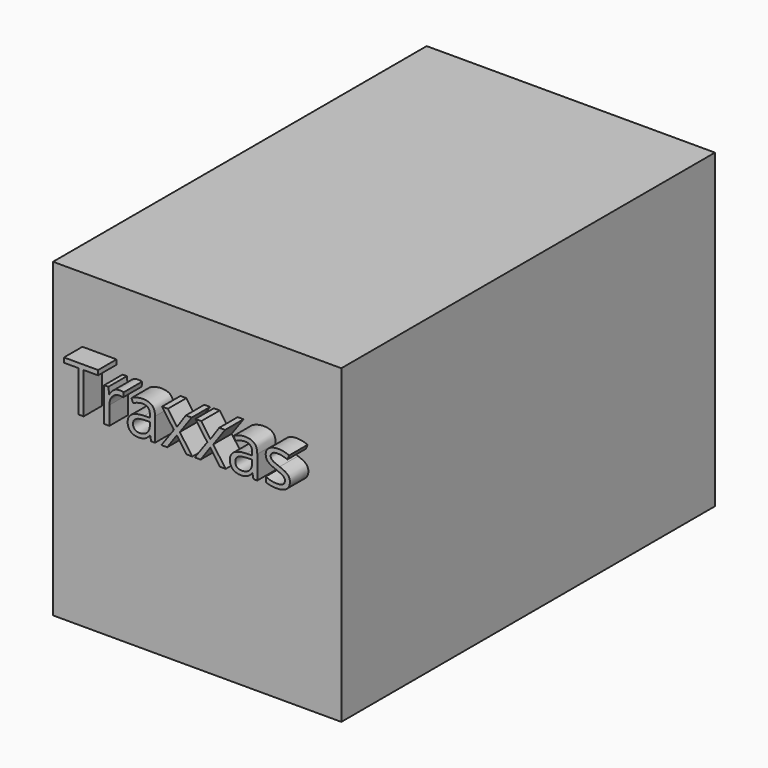
from build123d import *

# Parameters (mm, degrees)
F0_W         = 317.5
F0_H         = 342.9
F1_DEPTH     = 514.35
F2_TEXT_SIZE = 70.2142363511
F3_DEPTH     = 25.4


# Not quite as in the source:
# - Text() gives the source's letters only with a copy of the font that has no kerning and outlines rounded to 1/6400 em; it was checked with that copy


with BuildPart() as f1:
    # F0 (on Front) → F1 (new body)
    with BuildSketch(Plane.XZ):
        Rectangle(F0_W, F0_H)
    extrude(amount=F1_DEPTH)

    # F2 (on face) → F3 (join)
    with BuildSketch(Plane.XZ.offset(514.35)):
        with Locations((-127, 49.4038723482)):
            Text('Traxxas', F2_TEXT_SIZE, font='Open Sans', text_align=(TextAlign.LEFT, TextAlign.BOTTOM))
    extrude(amount=F3_DEPTH)


solid = f1.part
